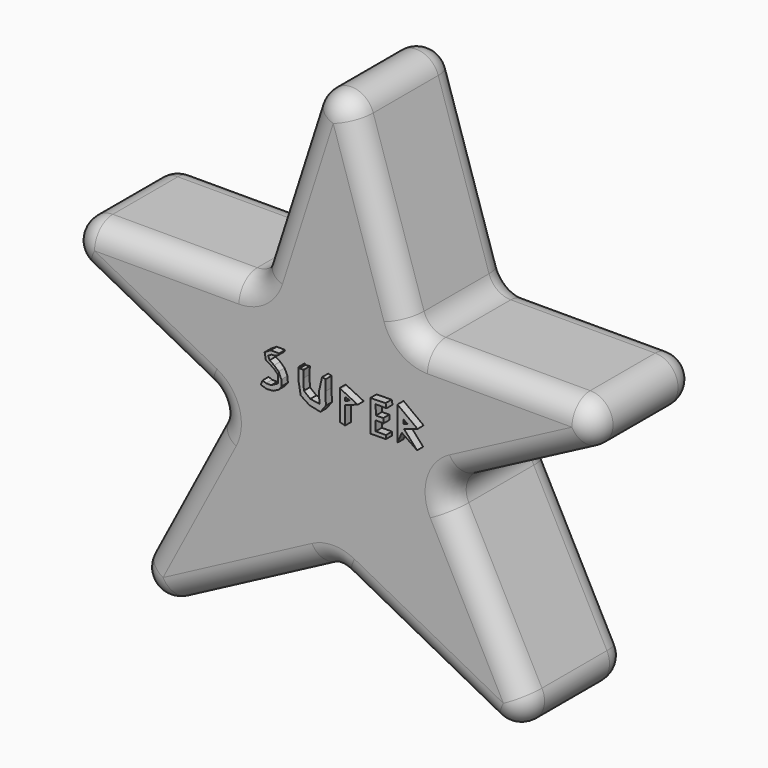
from build123d import *

# Parameters (mm, degrees)
F2_DEPTH = 6.35
F4_F1_R  = 2.286
F4_F2_R  = 2.286
F9_DEPTH = 0.762
F7_DEPTH = 0.762


with BuildPart() as f2:
    # F1 (on face) → F2 (new body, symmetric)
    with BuildSketch(Plane.XZ):
        Polygon((-22.4694542891, -22.4946287922), (0, -10.6504899906), (0, 35.9793268616), (-7.7678262384, 11.7962568429), (-33.1678262384, 11.7962568429), (-10.6731974462, 0), align=None)
    extrude(amount=F2_DEPTH, both=True)

    # F3: F2 across plane


with BuildPart() as f2_1:
    add(f2.part)
    add(f2.part.mirror(Plane.YZ))

    # F4: fillet of radius 2.286 on 26 edges, made by hand

    # F4_f1
    f4_f1_edges = [f2_1.edges().sort_by_distance(p)[0] for p in [
        (7.7678262384, 0, 11.7962568429),
        (10.6731974462, 0, 0),
        (0, 0, -10.6504899906),
        (-10.6731974462, 0, 0),
        (-7.7678262384, 0, 11.7962568429),
    ]]
    fillet(f4_f1_edges, radius=F4_F1_R)

    # F4_f2
    f4_f2_edges = [f2_1.edges().sort_by_distance(p)[0] for p in [
        (-11.7677133906, -6.35, -16.8535080516),
        (11.7677133906, -6.35, -16.8535080516),
        (17.1021574256, -6.35, -12.2595726917),
        (22.932770138, -6.35, 6.4289599794),
        (21.3012015954, -6.35, 11.7962568429),
        (3.6290503253, -6.35, 24.6812396715),
        (-3.6290503253, -6.35, 24.6812396715),
        (-21.3012015954, -6.35, 11.7962568429),
        (-22.932770138, -6.35, 6.4289599794),
        (-17.1021574256, -6.35, -12.2595726917),
        (0, 0, 35.9793268616),
        (3.6290503253, 6.35, 24.6812396715),
        (21.3012015954, 6.35, 11.7962568429),
        (33.1678262384, 0, 11.7962568429),
        (17.1021574256, 6.35, -12.2595726917),
        (22.4694542891, 0, -22.4946287922),
        (-11.7677133906, 6.35, -16.8535080516),
        (-22.4694542891, 0, -22.4946287922),
        (-22.932770138, 6.35, 6.4289599794),
        (-33.1678262384, 0, 11.7962568429),
        (-21.3012015954, 6.35, 11.7962568429),
        (-8.0877949674, 6.35, 12.2351038213),
        (-11.5771185545, 6.35, -0.2820132537),
        (0, 6.35, -10.948638197),
        (11.5771185545, 6.35, -0.2820132537),
        (8.0877949674, 6.35, 12.2351038213),
        (-11.5771185545, -6.35, -0.2820132537),
        (-8.0877949674, -6.35, 12.2351038213),
        (8.0877949674, -6.35, 12.2351038213),
        (11.5771185545, -6.35, -0.2820132537),
        (0, -6.35, -10.948638197),
    ]]
    fillet(f4_f2_edges, radius=F4_F2_R)

    # F8 (on face) → F9 (join)
    with BuildSketch(Plane.XZ.offset(6.35)):
        Polygon((-4.8077497631, 6.9738719612), (-4.8833619803, 6.9888005964), (-5.6563438848, 6.9888005964), (-6.2521840446, 6.6184131429), (-6.1394576915, 5.9903655201), (-5.3503718227, 5.4911477491), (-4.8953713849, 5.0424882211), (-4.8953713849, 4.3044914491), (-5.5958377197, 3.9264927618), (-6.1300005764, 3.9264927618), (-6.4605637453, 4.0734503418), (-6.6418400966, 3.6255908199), (-6.0233678669, 3.4443144687), (-5.4048956372, 3.4976312891), (-4.8717297614, 3.7642139941), (-4.5411670581, 4.180083517), (-4.583820235, 4.7665657476), (-4.8717297614, 5.3743747994), (-5.3089256398, 5.7795806788), (-5.7567846961, 6.078153383), (-5.9060710482, 6.4300429076), (-5.5541819893, 6.6433092579), (-5.223619286, 6.6433092579), (-4.9463729374, 6.7606056109), align=None)
    extrude(amount=F9_DEPTH)

    # F6 (on face) → F7 (join)
    with BuildSketch(Plane.XZ.offset(6.35)):
        Polygon((-2.7460011188, 6.3680754974), (-2.852873411, 6.4385421574), (-2.852873411, 5.140052177), (-2.6468993165, 3.9846990258), (-1.7563264119, 3.4034063574), (-0.6719225785, 3.1792041846), (-0.124490587, 3.912220709), (-0.1830757828, 5.1394319162), (-0.1522420207, 6.2248986214), (-0.5077649839, 6.2937401235), (-0.8040870307, 4.9930457026), (-0.7814072305, 3.8545557763), (-1.6878197202, 3.9909644984), (-2.3294347338, 4.5027183369), (-2.3874049075, 5.5876043625), (-2.337427577, 6.3529536128), (-2.7812926564, 6.314471364), align=None)
        Polygon((1.3429354876, 5.8594592847), (1.2765517458, 5.9258458205), (1.2765517458, 2.9113423079), (1.7961976118, 2.7786572464), (1.7949150642, 4.5979730785), (3.0550148804, 5.0231530331), align=None)
        Polygon((2.2798031569, 5.1395706832), (1.7628639471, 4.9090404063), (1.8159369938, 5.3025046363), align=None, mode=Mode.SUBTRACT)
        Polygon((5.8496114798, 6.0712443665), (4.3209996074, 6.0321558267), (4.3209996074, 4.947821144), (4.3456433341, 2.8858925216), (5.8767511191, 2.904191992), (5.8767511191, 3.2648150809), (4.8615592532, 3.2685473561), (4.8615592532, 4.235221073), (5.6510670111, 4.220648203), (5.6144981645, 4.6745948493), (4.8782676458, 4.666226916), (4.8519740812, 5.6559145451), (5.933160428, 5.6408806704), align=None)
        Polygon((7.0347818546, 6.3396086916), (7.0347818546, 2.9729763046), (7.4759777635, 3.9922273718), (9.0028224513, 2.937797457), (7.6884618029, 4.3934863061), (9.0492879972, 4.8372442834), align=None)
        Polygon((8.0597589084, 4.9393000391), (7.7467951924, 4.8372442834), (7.6166405343, 4.8372442834), (7.6166405343, 5.243926309), align=None, mode=Mode.SUBTRACT)
    extrude(amount=F7_DEPTH)


solid = f2_1.part
